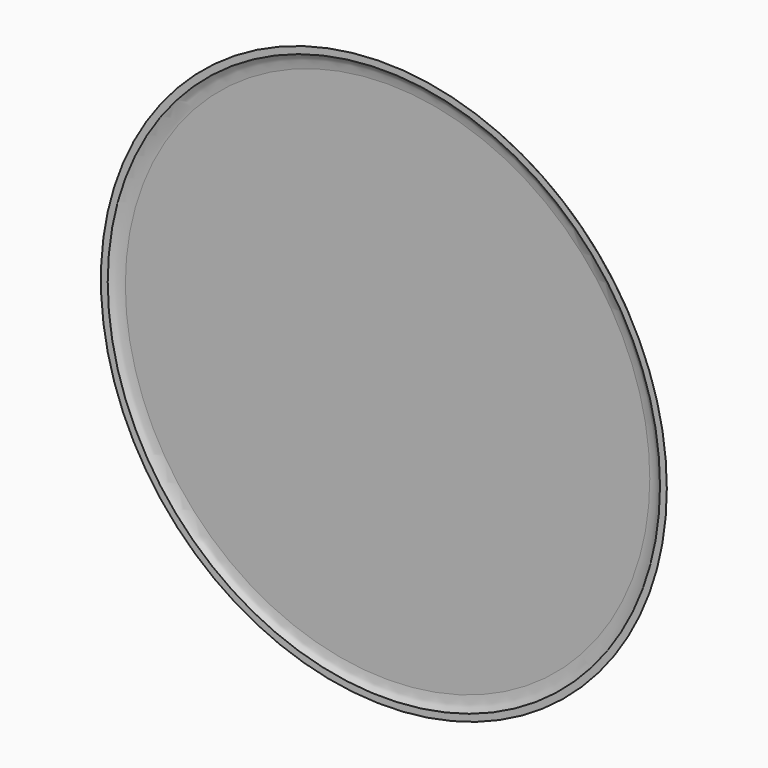
from build123d import *

# Parameters (mm, degrees)
F0_R     = 77.47
F1_DEPTH = 2.54
F3_T     = -1.27


# Not quite as in the source:
# - a fillet or chamfer that OpenCascade refuses, or shapes differently, is made with other operations: its cross-section is extruded or revolved along the edge and cut away or added
# - a feature names something its author has since deleted; it is built from what else it names


with BuildPart() as f1:
    # F0 (on Front) → F1 (new body)
    with BuildSketch(Plane.XZ):
        Circle(F0_R)
    extrude(amount=F1_DEPTH)

    # F2: fillet of radius 7.62 on 1 edges, made by hand

    # F2_s1 → F2_t2 (revolve, cut)
    with BuildSketch(Plane.XY):
        with BuildLine():
            ThreePointArc((77.47, -2.54), (74.9012393105, -0.6639235197), (71.7903873372, 0))
            Line((71.7903873372, 0), (77.47, 0))
            Line((77.47, 0), (77.47, -2.54))
        make_face()
    revolve(axis=Axis((0, 0, 0), (0, -1, 0)), mode=Mode.SUBTRACT)

    # F3
    f3_openings = [f1.faces().sort_by_distance(p)[0] for p in [
        (0, -2.54, 0),
    ]]
    offset(amount=F3_T, openings=f3_openings)


solid = f1.part
